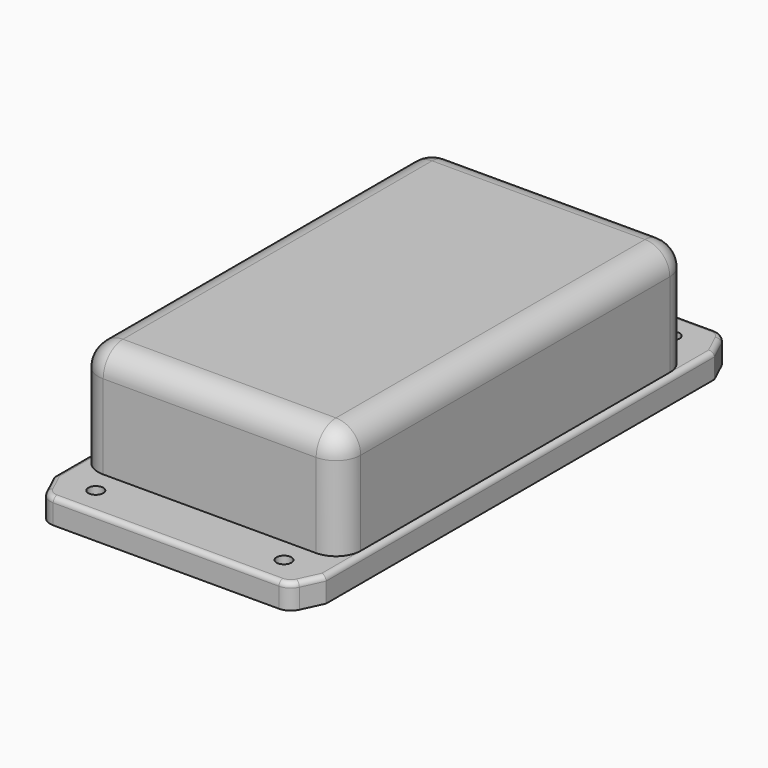
from build123d import *

# Parameters (mm, degrees)
F1_DEPTH = 5
F2_W     = 53
F2_H     = 88
F3_DEPTH = 22
F4_R     = 1.5
F5_DEPTH = 25
F6_R     = 5
F7_R     = 0.99999


# Not quite as in the source:
# - a fillet or chamfer is up to 0.001 mm smaller than in the source, because OpenCascade refuses the exact size


with BuildPart() as f1:
    # F0 (on Top) → F1 (new body)
    with BuildSketch(Plane.XY):
        with BuildLine():
            Line((22.7909432686, 55), (-22.7909432686, 55))
            ThreePointArc((-22.7909432686, 55), (-24.4028420937, 54.5301743374), (-25.5098666298, 53.2678547852))
            Line((-25.5098666298, 53.2678547852), (-27.5, 49))
            Line((-27.5, 49), (-27.5, -49))
            Line((-27.5, -49), (-25.5098666298, -53.2678547852))
            ThreePointArc((-25.5098666298, -53.2678547852), (-24.4028420937, -54.5301743374), (-22.7909432686, -55))
            Line((-22.7909432686, -55), (22.7909432686, -55))
            ThreePointArc((22.7909432686, -55), (24.4028420937, -54.5301743374), (25.5098666298, -53.2678547852))
            Line((25.5098666298, -53.2678547852), (27.5, -49))
            Line((27.5, -49), (27.5, 49))
            Line((27.5, 49), (25.5098666298, 53.2678547852))
            ThreePointArc((25.5098666298, 53.2678547852), (24.4028420937, 54.5301743374), (22.7909432686, 55))
        make_face()
    extrude(amount=F1_DEPTH)

    # F2 (on face) → F3 (join)
    with BuildSketch(Plane.XY.offset(5)):
        Rectangle(F2_W, F2_H)
    extrude(amount=F3_DEPTH)

    # F4 (on face) → F5 (cut)
    with BuildSketch(Plane.XY.offset(5)):
        with Locations((-19, 49)):
            Circle(F4_R)
        with Locations((19, 49)):
            Circle(F4_R)
        with Locations((-19, -49)):
            Circle(F4_R)
        with Locations((19, -49)):
            Circle(F4_R)
    extrude(amount=-F5_DEPTH, mode=Mode.SUBTRACT)

    # F6
    f6_edges = [f1.edges().sort_by_distance(p)[0] for p in [
        (-26.5, 0, 27),
        (0, 44, 27),
        (26.5, 0, 27),
        (0, -44, 27),
        (26.5, -44, 16),
        (26.5, 44, 16),
        (-26.5, 44, 16),
        (-26.5, -44, 16),
    ]]
    fillet(f6_edges, radius=F6_R)

    # F7 (radius 1 in the source; OpenCascade refuses exactly that, so slightly less here)
    f7_edges = [f1.edges().sort_by_distance(p)[0] for p in [
        (27.5, 0, 5),
        (26.504933, -51.133927, 5),
        (26.504933, 51.133927, 5),
        (-27.5, 0, 5),
    ]]
    fillet(f7_edges, radius=F7_R)


solid = f1.part
